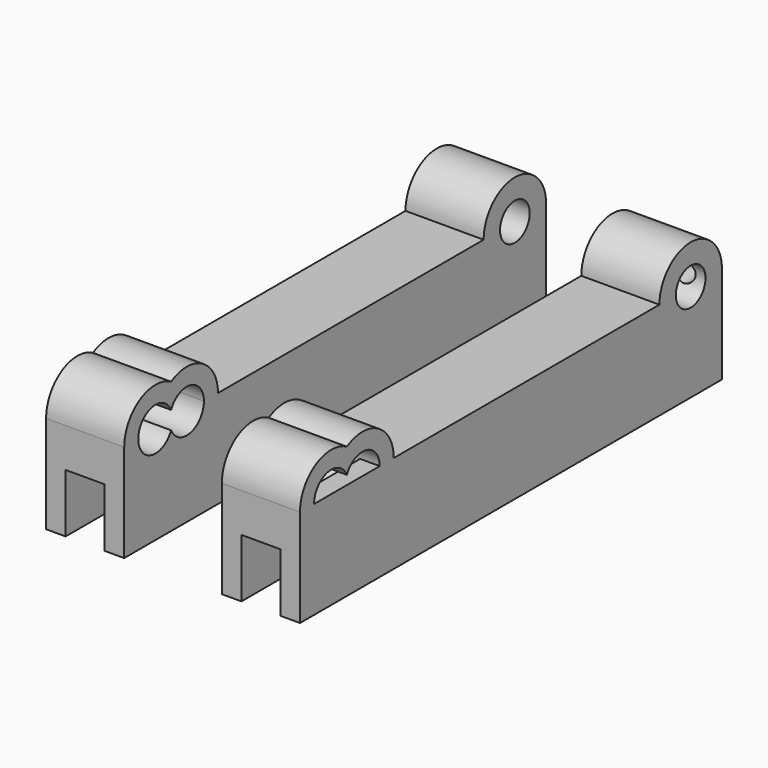
from build123d import *

# Parameters (mm, degrees)
F1_DEPTH  = 20
F0_W      = 135
F0_H      = 15
F2_DEPTH  = 5
F3_START  = 10
F2_FACE_W = 135
F2_FACE_H = 15
F3_DEPTH  = 5
F4_START  = 15
F4_DEPTH  = 5
F6_D      = 5
F6_DEPTH  = 12
F6_START  = 0.3175417
F6_TIP    = 1.5021515476


with BuildPart() as f1:
    # F0 (on Right) → F1 (new body)
    with BuildSketch(Plane.YZ):
        with BuildLine():
            ThreePointArc((-54.82459604, 6.7641116679), (-52.6360345491, 11.1555095091), (-47.81209604, 12.0520549117))
            ThreePointArc((-47.81209604, 12.0520549117), (-46.2759472816, 13.952902659), (-44.32459604, 15.4243657057))
            ThreePointArc((-44.32459604, 15.4243657057), (-54.32459604, 15.4243657057), (-59.32459604, 6.7641116679))
            Line((-59.32459604, 6.7641116679), (-54.82459604, 6.7641116679))
        make_face()
        with BuildLine():
            ThreePointArc((-40.83709604, 12.0520549117), (-36.0131575308, 11.1555095091), (-33.82459604, 6.7641116679))
            Line((-33.82459604, 6.7641116679), (-29.32459604, 6.7641116679))
            ThreePointArc((-29.32459604, 6.7641116679), (-34.32459604, 15.4243657057), (-44.32459604, 15.4243657057))
            ThreePointArc((-44.32459604, 15.4243657057), (-42.3732447983, 13.952902659), (-40.83709604, 12.0520549117))
        make_face()
        with BuildLine():
            ThreePointArc((-47.81209604, 12.0520549117), (-45.7401644318, 10.9356641422), (-44.32459604, 9.0553995153))
            ThreePointArc((-44.32459604, 9.0553995153), (-42.9090276481, 10.9356641422), (-40.83709604, 12.0520549117))
            ThreePointArc((-40.83709604, 12.0520549117), (-42.3732447983, 13.952902659), (-44.32459604, 15.4243657057))
            ThreePointArc((-44.32459604, 15.4243657057), (-46.2759472816, 13.952902659), (-47.81209604, 12.0520549117))
        make_face()
        with BuildLine():
            ThreePointArc((-33.82459604, 6.7641116679), (-38.1519921, 1.3905653528), (-44.32459604, 4.4728238204))
            ThreePointArc((-44.32459604, 4.4728238204), (-50.4971999799, 1.3905653528), (-54.82459604, 6.7641116679))
            Line((-54.82459604, 6.7641116679), (-59.32459604, 6.7641116679))
            Line((-59.32459604, 6.7641116679), (-59.32459604, -3.2358883321))
            Line((-59.32459604, -3.2358883321), (75.67540396, -3.2358883321))
            Line((75.67540396, -3.2358883321), (75.67540396, 6.7641116679))
            Line((75.67540396, 6.7641116679), (70.42540396, 6.7641116679))
            ThreePointArc((70.42540396, 6.7641116679), (65.67540396, 2.0141116679), (60.92540396, 6.7641116679))
            Line((60.92540396, 6.7641116679), (55.67540396, 6.7641116679))
            Line((55.67540396, 6.7641116679), (-29.32459604, 6.7641116679))
            Line((-29.32459604, 6.7641116679), (-33.82459604, 6.7641116679))
        make_face()
        with BuildLine():
            ThreePointArc((75.67540396, 6.7641116679), (65.67540396, 16.7641116679), (55.67540396, 6.7641116679))
            Line((55.67540396, 6.7641116679), (60.92540396, 6.7641116679))
            ThreePointArc((60.92540396, 6.7641116679), (65.67540396, 11.5141116679), (70.42540396, 6.7641116679))
            Line((70.42540396, 6.7641116679), (75.67540396, 6.7641116679))
        make_face()
    extrude(amount=F1_DEPTH)

    # F0 (on Right) → F2 (join)
    with BuildSketch(Plane.YZ):
        with Locations((8.17540396, -10.7358883321)):
            Rectangle(F0_W, F0_H)
    extrude(amount=F2_DEPTH)

    # F2_face (on face) → F3 (join)
    with BuildSketch(Plane(origin=(5, 8.17540396, -10.7358883321), x_dir=(0, 1, 0), z_dir=(1, 0, 0)).offset(F3_START)):
        Rectangle(F2_FACE_W, F2_FACE_H)
    extrude(amount=F3_DEPTH)

    # F0 (on Right) → F4 (join)
    with BuildSketch(Plane.YZ.offset(F4_START)):
        with BuildLine():
            ThreePointArc((-44.32459604, 4.4728238204), (-43.9510497249, 5.5915077279), (-43.82459604, 6.7641116679))
            Line((-43.82459604, 6.7641116679), (-44.82459604, 6.7641116679))
            ThreePointArc((-44.82459604, 6.7641116679), (-44.698142355, 5.5915077279), (-44.32459604, 4.4728238204))
        make_face()
        with BuildLine():
            Line((-39.32459604, 6.7641116679), (-43.82459604, 6.7641116679))
            ThreePointArc((-43.82459604, 6.7641116679), (-43.9510497249, 5.5915077279), (-44.32459604, 4.4728238204))
            ThreePointArc((-44.32459604, 4.4728238204), (-38.1519921, 1.3905653528), (-33.82459604, 6.7641116679))
            Line((-33.82459604, 6.7641116679), (-39.32459604, 6.7641116679))
        make_face()
        with BuildLine():
            ThreePointArc((-44.32459604, 4.4728238204), (-44.698142355, 5.5915077279), (-44.82459604, 6.7641116679))
            Line((-44.82459604, 6.7641116679), (-49.32459604, 6.7641116679))
            Line((-49.32459604, 6.7641116679), (-54.82459604, 6.7641116679))
            ThreePointArc((-54.82459604, 6.7641116679), (-50.4971999799, 1.3905653528), (-44.32459604, 4.4728238204))
        make_face()
        with BuildLine():
            ThreePointArc((-33.82459604, 6.7641116679), (-38.1519921, 1.3905653528), (-44.32459604, 4.4728238204))
            ThreePointArc((-44.32459604, 4.4728238204), (-50.4971999799, 1.3905653528), (-54.82459604, 6.7641116679))
            Line((-54.82459604, 6.7641116679), (-59.32459604, 6.7641116679))
            Line((-59.32459604, 6.7641116679), (-59.32459604, -3.2358883321))
            Line((-59.32459604, -3.2358883321), (75.67540396, -3.2358883321))
            Line((75.67540396, -3.2358883321), (75.67540396, 6.7641116679))
            Line((75.67540396, 6.7641116679), (70.42540396, 6.7641116679))
            ThreePointArc((70.42540396, 6.7641116679), (65.67540396, 2.0141116679), (60.92540396, 6.7641116679))
            Line((60.92540396, 6.7641116679), (55.67540396, 6.7641116679))
            Line((55.67540396, 6.7641116679), (-29.32459604, 6.7641116679))
            Line((-29.32459604, 6.7641116679), (-33.82459604, 6.7641116679))
        make_face()
    extrude(amount=F4_DEPTH)

    # F6
    # its depths count from where the whole tool has entered the part; down to there all is cleared
    with Locations(Plane(origin=(0, 75.67540396, 0), x_dir=(-1, 0, 0), z_dir=(0, 1, 0)).offset(-F6_START)):
        with Locations((-15, 6.7641116679)):
            Hole(F6_D / 2, depth=F6_DEPTH)
            with Locations((0, 0, -(F6_DEPTH + F6_TIP / 2))):  # 118° drill point
                Cone(0, F6_D / 2, F6_TIP, mode=Mode.SUBTRACT)


with BuildPart() as f7_1:
    # F7: instance of F1
    add(f1.part.mirror(Plane.YZ))


with BuildPart() as f7_1_1:
    # F8: moved
    add(f7_1.part.moved(Location((-25, 0, 0))))


solid = Compound([f1.part, f7_1_1.part])
